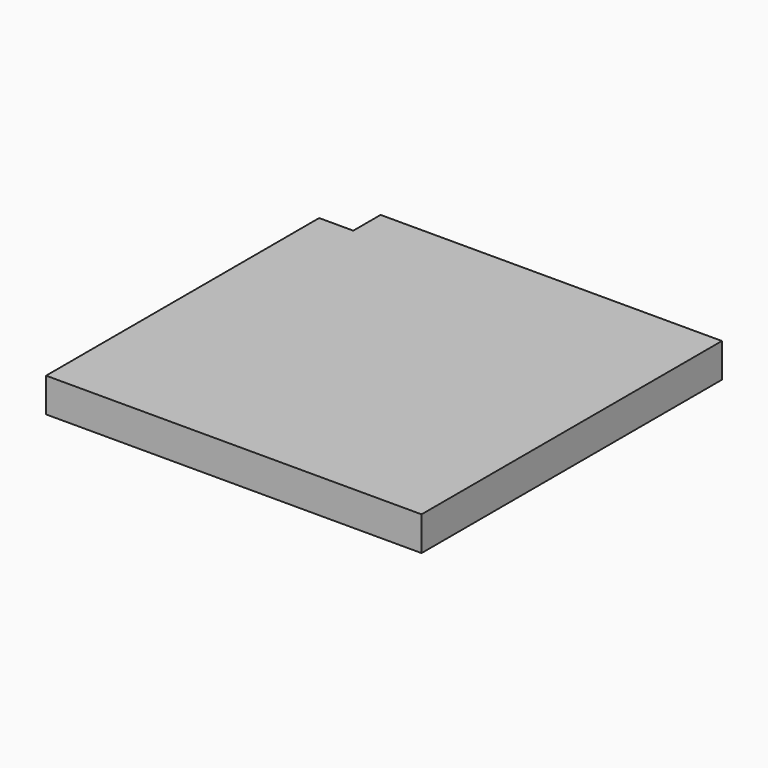
from build123d import *

# Parameters (mm, degrees)
F0_W     = 31.75
F0_H     = 31.75
F1_DEPTH = 3.175
F2_W     = 31.75
F2_H     = 3.175
F3_DEPTH = 3.175
F4_W     = 3.175
F4_H     = 31.75
F5_DEPTH = 3.175


# Not quite as in the source:
# - a length typed as a fraction of an inch, garbled in the dataset ("3 / 203.2 mm" for 3/8 in), is restored


with BuildPart() as f1:
    # F0 (on Top) → F1 (new body)
    with BuildSketch(Plane.XY):
        Rectangle(F0_W, F0_H)
    extrude(amount=F1_DEPTH)

    # F2 (on face) → F3 (join)
    with BuildSketch(Plane.XY.offset(3.175)):
        with Locations((0, 17.4625)):
            Rectangle(F2_W, F2_H)
    extrude(amount=-F3_DEPTH)

    # F4 (on face) → F5 (join)
    with BuildSketch(Plane.XY.offset(3.175)):
        with Locations((-17.4625, 0)):
            Rectangle(F4_W, F4_H)
    extrude(amount=-F5_DEPTH)


solid = f1.part
